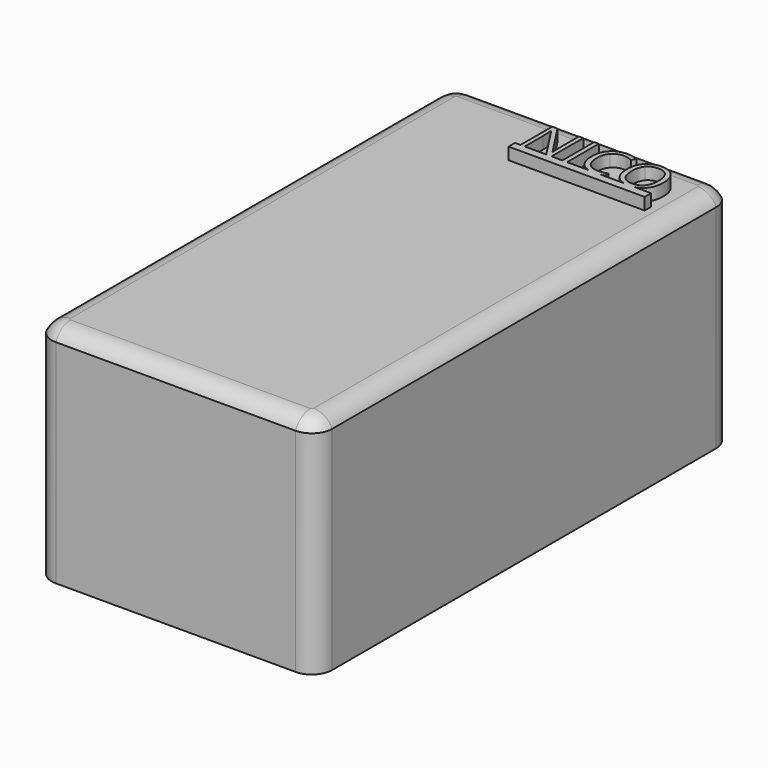
from build123d import *

# Parameters (mm, degrees)
F0_W          = 70
F0_H          = 130
F0_W_2        = 64
F0_H_2        = 124
F1_DEPTH      = 50
F2_W          = 70
F2_H          = 3
F3_DEPTH      = 130
F4_R          = 5.08
F5_R          = 5.08
F7_DEPTH      = 3
F8_W          = 70
F8_H          = 130
F9_DEPTH      = 3
F10_R         = 5.08
F11_W         = 1.15234375
F11_H         = 9.9153645833
F12_DEPTH     = 3
F13_T1_DEPTH  = 59.84
F13_T3_DEPTH  = 119.84
F13_T6_ANGLE  = 90
F13_T8_ANGLE  = 90
F13_T10_ANGLE = 90
F13_T12_ANGLE = 90


# Not quite as in the source:
# - a fillet or chamfer that OpenCascade refuses, or shapes differently, is made with other operations: its cross-section is extruded or revolved along the edge and cut away or added


with BuildPart() as f1:
    # F0 (on Top) → F1 (new body)
    with BuildSketch(Plane.XY):
        Rectangle(F0_W, F0_H)
        Rectangle(F0_W_2, F0_H_2, mode=Mode.SUBTRACT)
    extrude(amount=F1_DEPTH)

    # F2 (on face) → F3 (join, through all)
    with BuildSketch(Plane.XZ.offset(65)):
        with Locations((0, -1.5)):
            Rectangle(F2_W, F2_H)
    extrude(amount=-F3_DEPTH)

    # F4
    f4_edges = [f1.edges().sort_by_distance(p)[0] for p in [
        (35, 65, 23.5),
        (-35, 65, 23.5),
        (-35, -65, 23.5),
        (35, -65, 23.5),
    ]]
    fillet(f4_edges, radius=F4_R)

    # F5
    f5_edges = [f1.edges().sort_by_distance(p)[0] for p in [
        (-32, -62, 25),
        (-32, 62, 25),
        (32, 62, 25),
        (32, -62, 25),
    ]]
    fillet(f5_edges, radius=F5_R)


with BuildPart() as f7:
    # F6 (on face) → F7 (new body)
    with BuildSketch(Plane.XY.offset(50)):
        with BuildLine():
            Line((26.92, 62), (-26.92, 62))
            ThreePointArc((-26.92, 62), (-30.5121024484, 60.5121024484), (-32, 56.92))
            Line((-32, 56.92), (-32, -56.92))
            ThreePointArc((-32, -56.92), (-30.5121024484, -60.5121024484), (-26.92, -62))
            Line((-26.92, -62), (26.92, -62))
            ThreePointArc((26.92, -62), (30.5121024484, -60.5121024484), (32, -56.92))
            Line((32, -56.92), (32, 56.92))
            ThreePointArc((32, 56.92), (30.5121024484, 60.5121024484), (26.92, 62))
        make_face()
    extrude(amount=-F7_DEPTH)

    # F8 (on face) → F9 (join)
    with BuildSketch(Plane.XY.offset(50)):
        Rectangle(F8_W, F8_H)
    extrude(amount=F9_DEPTH)

    # F10
    f10_edges = [f7.edges().sort_by_distance(p)[0] for p in [
        (-35, 65, 51.5),
        (-35, -65, 51.5),
        (35, -65, 51.5),
        (35, 65, 51.5),
    ]]
    fillet(f10_edges, radius=F10_R)

    # F13: fillet of radius 5.08 on 1 edges, made by hand

    # F13_s2 → F13_t1 (cut)
    with BuildSketch(Plane.YZ.offset(-29.92)):
        with BuildLine():
            ThreePointArc((-60.3653479095, 53), (-63.1257826579, 52.1845515591), (-65, 50))
            Line((-65, 50), (-65, 53))
            Line((-65, 53), (-60.3653479095, 53))
        make_face()
        with BuildLine():
            ThreePointArc((65, 50), (63.1257826579, 52.1845515591), (60.3653479095, 53))
            Line((60.3653479095, 53), (65, 53))
            Line((65, 53), (65, 50))
        make_face()
    extrude(amount=F13_T1_DEPTH, mode=Mode.SUBTRACT)

    # F13_s4 → F13_t3 (cut)
    with BuildSketch(Plane.XZ.offset(-59.92)):
        with BuildLine():
            ThreePointArc((30.3653479095, 53), (33.1257826579, 52.1845515591), (35, 50))
            Line((35, 50), (35, 53))
            Line((35, 53), (30.3653479095, 53))
        make_face()
        with BuildLine():
            ThreePointArc((-30.3653479095, 53), (-33.1257826579, 52.1845515591), (-35, 50))
            Line((-35, 50), (-35, 53))
            Line((-35, 53), (-30.3653479095, 53))
        make_face()
    extrude(amount=F13_T3_DEPTH, mode=Mode.SUBTRACT)

    # F13_s5 → F13_t6 (revolve, cut)
    with BuildSketch(Plane.XZ.offset(59.92)):
        with BuildLine():
            ThreePointArc((-30.3653479095, 53), (-33.1257826579, 52.1845515591), (-35, 50))
            Line((-35, 50), (-35, 53))
            Line((-35, 53), (-30.3653479095, 53))
        make_face()
    revolve(axis=Axis((-29.92, -59.92, 53), (0, 0, 1)), revolution_arc=F13_T6_ANGLE, mode=Mode.SUBTRACT)

    # F13_s7 → F13_t8 (revolve, cut)
    with BuildSketch(Plane.XZ.offset(59.92)):
        with BuildLine():
            ThreePointArc((30.3653479095, 53), (33.1257826579, 52.1845515591), (35, 50))
            Line((35, 50), (35, 53))
            Line((35, 53), (30.3653479095, 53))
        make_face()
    revolve(axis=Axis((29.92, -59.92, 53), (0, 0, -1)), revolution_arc=F13_T8_ANGLE, mode=Mode.SUBTRACT)

    # F13_s9 → F13_t10 (revolve, cut)
    with BuildSketch(Plane.YZ.offset(29.92)):
        with BuildLine():
            ThreePointArc((65, 50), (63.1257826579, 52.1845515591), (60.3653479095, 53))
            Line((60.3653479095, 53), (65, 53))
            Line((65, 53), (65, 50))
        make_face()
    revolve(axis=Axis((29.92, 59.92, 53), (0, 0, -1)), revolution_arc=F13_T10_ANGLE, mode=Mode.SUBTRACT)

    # F13_s11 → F13_t12 (revolve, cut)
    with BuildSketch(Plane.YZ.offset(-29.92)):
        with BuildLine():
            ThreePointArc((65, 50), (63.1257826579, 52.1845515591), (60.3653479095, 53))
            Line((60.3653479095, 53), (65, 53))
            Line((65, 53), (65, 50))
        make_face()
    revolve(axis=Axis((-29.92, 59.92, 53), (0, 0, 1)), revolution_arc=F13_T12_ANGLE, mode=Mode.SUBTRACT)


with BuildPart() as f12:
    # F11 (on face) → F12 (new body)
    with BuildSketch(Plane.XY.offset(53)):
        with BuildLine():
            Line((-4.0095031147, 47.5973086248), (-5.3723503369, 47.5973086248))
            Line((-5.3723503369, 47.5973086248), (-5.3723503369, 45.5973086248))
            Line((-5.3723503369, 45.5973086248), (28.6033441075, 45.5973086248))
            Line((28.6033441075, 45.5973086248), (28.6033441075, 47.5973086248))
            Line((28.6033441075, 47.5973086248), (24.414270697, 47.5973086248))
            add(Edge.make_bspline(
                [(24.414270697, 47.5973086248), (23.8300998313, 47.4605898748), (23.1519552187, 47.4605898748)],
                knots=[0.6833950988, 0.6833950988, 0.6833950988, 1, 1, 1], degree=2))
            add(Edge.make_bspline(
                [(23.1519552187, 47.4605898748), (22.4525473893, 47.4605898748), (21.8550974295, 47.5973086248)],
                knots=[0, 0, 0, 0.319412416, 0.319412416, 0.319412416], degree=2))
            Line((21.8550974295, 47.5973086248), (16.0140816741, 47.5973086248))
            add(Edge.make_bspline(
                [(16.0140816741, 47.5973086248), (15.2862889306, 47.4605898748), (14.3889343853, 47.4605898748)],
                knots=[0.406741787, 0.406741787, 0.406741787, 1, 1, 1], degree=2))
            add(Edge.make_bspline(
                [(14.3889343853, 47.4605898748), (13.6869640925, 47.4605898748), (13.0877001364, 47.5973086248)],
                knots=[0, 0, 0, 0.3205826669, 0.3205826669, 0.3205826669], degree=2))
            Line((13.0877001364, 47.5973086248), (7.6137607742, 47.5973086248))
            Line((7.6137607742, 47.5973086248), (6.4614170242, 47.5973086248))
            Line((6.4614170242, 47.5973086248), (3.7357225798, 47.5973086248))
            Line((3.7357225798, 47.5973086248), (2.4206184131, 47.5973086248))
            Line((2.4206184131, 47.5973086248), (-2.9439649202, 47.5973086248))
            Line((-2.9439649202, 47.5973086248), (-4.0095031147, 47.5973086248))
        make_face()
        with BuildLine():
            Line((-4.0095031147, 57.5126732081), (-4.0095031147, 47.5973086248))
            Line((-4.0095031147, 47.5973086248), (-2.9439649202, 47.5973086248))
            Line((-2.9439649202, 47.5973086248), (-2.9439649202, 53.2331593192))
            add(Edge.make_bspline(
                [(-3.0524718647, 55.9176211248), (-2.9439649202, 54.4527773748), (-2.9439649202, 53.2331593192)],
                knots=[0, 0, 0, 1, 1, 1], degree=2))
            Line((-3.0524718647, 55.9176211248), (-2.9982183925, 55.9176211248))
            Line((-2.9982183925, 55.9176211248), (2.4206184131, 47.5973086248))
            Line((2.4206184131, 47.5973086248), (3.7357225798, 47.5973086248))
            Line((3.7357225798, 47.5973086248), (3.7357225798, 57.5126732081))
            Line((3.7357225798, 57.5126732081), (2.657163552, 57.5126732081))
            Line((2.657163552, 57.5126732081), (2.657163552, 51.8225690414))
            add(Edge.make_bspline(
                [(2.6918857742, 50.4011280692), (2.6441427187, 51.3950516803), (2.657163552, 51.8225690414)],
                knots=[0, 0, 0, 1, 1, 1], degree=2))
            add(Edge.make_bspline(
                [(2.7526496631, 49.2249127914), (2.7396288298, 49.4072044581), (2.6918857742, 50.4011280692)],
                knots=[0, 0, 0, 1, 1, 1], degree=2))
            Line((2.7526496631, 49.2249127914), (2.6983961909, 49.2249127914))
            Line((2.6983961909, 49.2249127914), (-2.7074197813, 57.5126732081))
            Line((-2.7074197813, 57.5126732081), (-4.0095031147, 57.5126732081))
        make_face()
        with BuildLine():
            add(Edge.make_bspline(
                [(24.414270697, 47.5973086248), (23.8300998313, 47.4605898748), (23.1519552187, 47.4605898748)],
                knots=[0.6833950988, 0.6833950988, 0.6833950988, 1, 1, 1], degree=2))
            Line((24.414270697, 47.5973086248), (21.8550974295, 47.5973086248))
            add(Edge.make_bspline(
                [(23.1519552187, 47.4605898748), (22.4525473893, 47.4605898748), (21.8550974295, 47.5973086248)],
                knots=[0, 0, 0, 0.319412416, 0.319412416, 0.319412416], degree=2))
        make_face()
        with BuildLine():
            Line((21.8550974295, 47.5973086248), (24.414270697, 47.5973086248))
            add(Edge.make_bspline(
                [(26.4983093853, 48.8245221664), (25.6752098198, 47.8924175233), (24.414270697, 47.5973086248)],
                knots=[0, 0, 0, 0.6833950988, 0.6833950988, 0.6833950988], degree=2))
            add(Edge.make_bspline(
                [(27.7027364687, 52.5690968192), (27.7027364687, 50.1884544581), (26.4983093853, 48.8245221664)],
                knots=[0, 0, 0, 1, 1, 1], degree=2))
            add(Edge.make_bspline(
                [(26.5026496631, 56.3125864026), (27.7027364687, 54.956249597), (27.7027364687, 52.5690968192)],
                knots=[0, 0, 0, 1, 1, 1], degree=2))
            add(Edge.make_bspline(
                [(23.164976052, 57.6689232081), (25.3025628575, 57.6689232081), (26.5026496631, 56.3125864026)],
                knots=[0, 0, 0, 1, 1, 1], degree=2))
            add(Edge.make_bspline(
                [(19.7752191075, 56.3364579303), (20.9687954964, 57.6689232081), (23.164976052, 57.6689232081)],
                knots=[0, 0, 0, 1, 1, 1], degree=2))
            add(Edge.make_bspline(
                [(18.5816427187, 52.5821176526), (18.5816427187, 55.0039926526), (19.7752191075, 56.3364579303)],
                knots=[0, 0, 0, 1, 1, 1], degree=2))
            add(Edge.make_bspline(
                [(19.7719638992, 48.8006506387), (18.5816427187, 50.1407114026), (18.5816427187, 52.5821176526)],
                knots=[0, 0, 0, 1, 1, 1], degree=2))
            add(Edge.make_bspline(
                [(21.8550974295, 47.5973086248), (20.5820817157, 47.888621921), (19.7719638992, 48.8006506387)],
                knots=[0.319412416, 0.319412416, 0.319412416, 1, 1, 1], degree=2))
        make_face()
        with BuildLine():
            add(Edge.make_bspline(
                [(19.8012607742, 52.5690968192), (19.8012607742, 50.5552079303), (20.6595507048, 49.5135412637)],
                knots=[0, 0, 0, 1, 1, 1], degree=2))
            add(Edge.make_bspline(
                [(20.6595507048, 55.5964405692), (19.8012607742, 54.5547739026), (19.8012607742, 52.5690968192)],
                knots=[0, 0, 0, 1, 1, 1], degree=2))
            add(Edge.make_bspline(
                [(23.164976052, 56.6381072359), (21.5178406353, 56.6381072359), (20.6595507048, 55.5964405692)],
                knots=[0, 0, 0, 1, 1, 1], degree=2))
            add(Edge.make_bspline(
                [(25.6432746631, 55.6040360553), (24.805601052, 56.6381072359), (23.164976052, 56.6381072359)],
                knots=[0, 0, 0, 1, 1, 1], degree=2))
            add(Edge.make_bspline(
                [(26.4809482742, 52.5690968192), (26.4809482742, 54.5699648748), (25.6432746631, 55.6040360553)],
                knots=[0, 0, 0, 1, 1, 1], degree=2))
            add(Edge.make_bspline(
                [(25.6400194548, 49.5092009859), (26.4809482742, 50.5465273748), (26.4809482742, 52.5690968192)],
                knots=[0, 0, 0, 1, 1, 1], degree=2))
            add(Edge.make_bspline(
                [(23.1519552187, 48.471874597), (24.7990906353, 48.471874597), (25.6400194548, 49.5092009859)],
                knots=[0, 0, 0, 1, 1, 1], degree=2))
            add(Edge.make_bspline(
                [(20.6595507048, 49.5135412637), (21.5178406353, 48.471874597), (23.1519552187, 48.471874597)],
                knots=[0, 0, 0, 1, 1, 1], degree=2))
        make_face(mode=Mode.SUBTRACT)
        with Locations((7.0375888992, 52.5549909164)):
            Rectangle(F11_W, F11_H)
        with BuildLine():
            add(Edge.make_bspline(
                [(16.0140816741, 47.5973086248), (15.2862889306, 47.4605898748), (14.3889343853, 47.4605898748)],
                knots=[0.406741787, 0.406741787, 0.406741787, 1, 1, 1], degree=2))
            Line((16.0140816741, 47.5973086248), (13.0877001364, 47.5973086248))
            add(Edge.make_bspline(
                [(14.3889343853, 47.4605898748), (13.6869640925, 47.4605898748), (13.0877001364, 47.5973086248)],
                knots=[0, 0, 0, 0.3205826669, 0.3205826669, 0.3205826669], degree=2))
        make_face()
        with BuildLine():
            Line((13.0877001364, 47.5973086248), (16.0140816741, 47.5973086248))
            add(Edge.make_bspline(
                [(16.9323371631, 47.8490447359), (16.5130612325, 47.6910439115), (16.0140816741, 47.5973086248)],
                knots=[0, 0, 0, 0.406741787, 0.406741787, 0.406741787], degree=2))
            Line((16.9323371631, 47.8490447359), (16.9323371631, 48.8581593192))
            add(Edge.make_bspline(
                [(14.5647156353, 48.4848954303), (15.6020420242, 48.4848954303), (16.9323371631, 48.8581593192)],
                knots=[0, 0, 0, 1, 1, 1], degree=2))
            add(Edge.make_bspline(
                [(11.963804177, 49.5471784164), (12.8763475798, 48.4848954303), (14.5647156353, 48.4848954303)],
                knots=[0, 0, 0, 1, 1, 1], degree=2))
            add(Edge.make_bspline(
                [(11.0512607742, 52.553905847), (11.0512607742, 50.6094614026), (11.963804177, 49.5471784164)],
                knots=[0, 0, 0, 1, 1, 1], degree=2))
            add(Edge.make_bspline(
                [(11.9974413298, 55.5345916109), (11.0512607742, 54.4462669581), (11.0512607742, 52.553905847)],
                knots=[0, 0, 0, 1, 1, 1], degree=2))
            add(Edge.make_bspline(
                [(14.5777364687, 56.6229162637), (12.9436218853, 56.6229162637), (11.9974413298, 55.5345916109)],
                knots=[0, 0, 0, 1, 1, 1], degree=2))
            add(Edge.make_bspline(
                [(16.8303406353, 56.0955725137), (15.704038552, 56.6229162637), (14.5777364687, 56.6229162637)],
                knots=[0, 0, 0, 1, 1, 1], degree=2))
            Line((16.8303406353, 56.0955725137), (17.3186218853, 57.085155847))
            add(Edge.make_bspline(
                [(14.5929274409, 57.6537322359), (16.1510871631, 57.6537322359), (17.3186218853, 57.085155847)],
                knots=[0, 0, 0, 1, 1, 1], degree=2))
            add(Edge.make_bspline(
                [(12.0462694548, 57.0298173053), (13.1280836909, 57.6537322359), (14.5929274409, 57.6537322359)],
                knots=[0, 0, 0, 1, 1, 1], degree=2))
            add(Edge.make_bspline(
                [(10.391538552, 55.2535586248), (10.9644552187, 56.4059023748), (12.0462694548, 57.0298173053)],
                knots=[0, 0, 0, 1, 1, 1], degree=2))
            add(Edge.make_bspline(
                [(9.8186218853, 52.5690968192), (9.8186218853, 54.1012148748), (10.391538552, 55.2535586248)],
                knots=[0, 0, 0, 1, 1, 1], degree=2))
            add(Edge.make_bspline(
                [(11.0089430659, 48.7908850137), (9.8186218853, 50.1211801526), (9.8186218853, 52.5690968192)],
                knots=[0, 0, 0, 1, 1, 1], degree=2))
            add(Edge.make_bspline(
                [(13.0877001364, 47.5973086248), (11.8176679079, 47.8870594382), (11.0089430659, 48.7908850137)],
                knots=[0.3205826669, 0.3205826669, 0.3205826669, 1, 1, 1], degree=2))
        make_face()
    extrude(amount=F12_DEPTH)


solid = Compound([f1.part, f7.part, f12.part])
